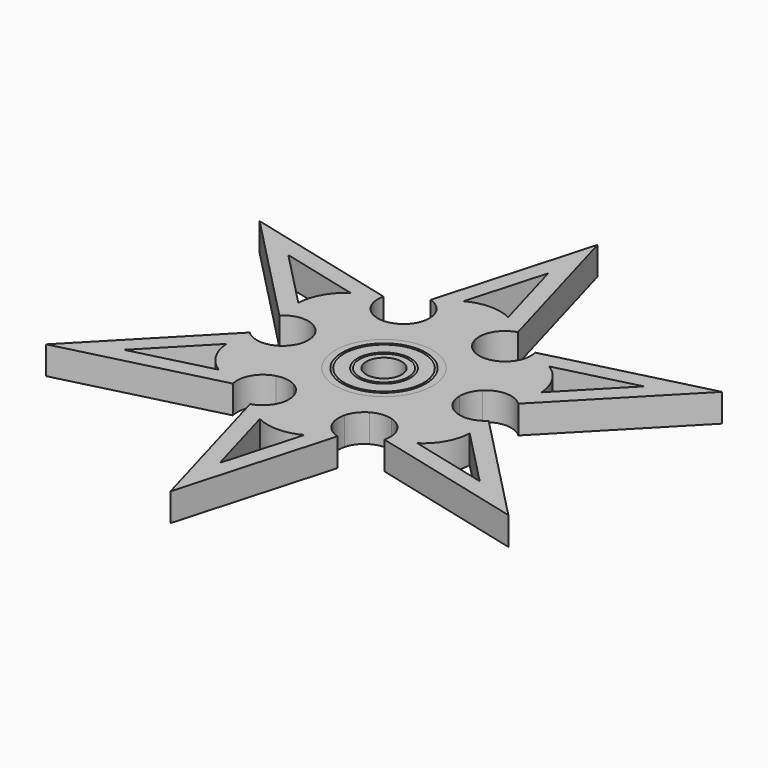
from build123d import *

# Parameters (mm, degrees)
F1_R     = 11
F1_R_2   = 4
F2_DEPTH = 6.35
F5_R     = 11
F6_DEPTH = 6.35
F8_DEPTH = 25.4


with BuildPart() as f2:
    # F1 (on Top) → F2 (new body)
    with BuildSketch(Plane.XY):
        Circle(F1_R)
        Circle(F1_R_2, mode=Mode.SUBTRACT)
    extrude(amount=F2_DEPTH)

    # F3 (on Right) → F4 (revolve, cut)
    with BuildSketch(Plane.YZ):
        with BuildLine():
            ThreePointArc((6, 6.35), (5.75, 6.6), (5.5, 6.35))
            Line((5.5, 6.35), (5.75, 6.35))
            Line((5.75, 6.35), (6, 6.35))
        make_face()
        with BuildLine():
            ThreePointArc((9.5, 6.35), (9.25, 6.6), (9, 6.35))
            Line((9, 6.35), (9.25, 6.35))
            Line((9.25, 6.35), (9.5, 6.35))
        make_face()
        with BuildLine():
            Line((9.25, 6.35), (9, 6.35))
            ThreePointArc((9, 6.35), (9.25, 6.1), (9.5, 6.35))
            Line((9.5, 6.35), (9.25, 6.35))
        make_face()
        with BuildLine():
            Line((5.75, 6.35), (5.5, 6.35))
            ThreePointArc((5.5, 6.35), (5.75, 6.1), (6, 6.35))
            Line((6, 6.35), (5.75, 6.35))
        make_face()
    revolve(axis=Axis((0, 0, 3.175), (0, 0, 1)), mode=Mode.SUBTRACT)


with BuildPart() as f6:
    # F5 (on Top) → F6 (new body)
    with BuildSketch(Plane.XY):
        with BuildLine():
            Line((0, 60.5), (0, 17.0180425354))
            Line((0, 17.0180425354), (5.8258503254, 18.4893295859))
            ThreePointArc((5.8258503254, 18.4893295859), (6.4320296551, 22.8503868027), (9.9057263273, 25.5558821098))
            Line((9.9057263273, 25.5558821098), (0, 60.5))
        make_face()
        with BuildLine():
            Line((-5.8258503254, 18.4893295859), (0, 17.0180425354))
            Line((0, 17.0180425354), (0, 60.5))
            Line((0, 60.5), (-9.9057263273, 25.5558821098))
            ThreePointArc((-9.9057263273, 25.5558821098), (-6.4320296551, 22.8503868027), (-5.8258503254, 18.4893295859))
        make_face()
        with BuildLine():
            Line((-18.9251542831, 4.1993304125), (-14.7380571583, 8.5090212677))
            Line((-14.7380571583, 8.5090212677), (-13.0993039576, 14.2899991734))
            ThreePointArc((-13.0993039576, 14.2899991734), (-16.5730006299, 16.9954944805), (-17.1791799596, 21.3565516973))
            Line((-17.1791799596, 21.3565516973), (-52.394536929, 30.25))
            Line((-52.394536929, 30.25), (-27.0849062869, 4.1993304125))
            ThreePointArc((-27.0849062869, 4.1993304125), (-23.005030285, 5.8548923222), (-18.9251542831, 4.1993304125))
        make_face()
        with BuildLine():
            Line((-13.0993039576, -14.2899991734), (-14.7380571583, -8.5090212677))
            Line((-14.7380571583, -8.5090212677), (-18.9251542831, -4.1993304125))
            ThreePointArc((-18.9251542831, -4.1993304125), (-23.005030285, -5.8548923222), (-27.0849062869, -4.1993304125))
            Line((-27.0849062869, -4.1993304125), (-52.394536929, -30.25))
            Line((-52.394536929, -30.25), (-17.1791799596, -21.3565516973))
            ThreePointArc((-17.1791799596, -21.3565516973), (-16.5730006299, -16.9954944805), (-13.0993039576, -14.2899991734))
        make_face()
        with BuildLine():
            Line((5.8258503254, -18.4893295859), (0, -17.0180425354))
            Line((0, -17.0180425354), (-5.8258503254, -18.4893295859))
            ThreePointArc((-5.8258503254, -18.4893295859), (-6.4320296551, -22.8503868027), (-9.9057263273, -25.5558821098))
            Line((-9.9057263273, -25.5558821098), (0, -60.5))
            Line((0, -60.5), (9.9057263273, -25.5558821098))
            ThreePointArc((9.9057263273, -25.5558821098), (6.4320296551, -22.8503868027), (5.8258503254, -18.4893295859))
        make_face()
        with BuildLine():
            Line((18.9251542831, -4.1993304125), (14.7380571583, -8.5090212677))
            Line((14.7380571583, -8.5090212677), (13.0993039576, -14.2899991734))
            ThreePointArc((13.0993039576, -14.2899991734), (16.5730006299, -16.9954944805), (17.1791799596, -21.3565516973))
            Line((17.1791799596, -21.3565516973), (52.394536929, -30.25))
            Line((52.394536929, -30.25), (27.0849062869, -4.1993304125))
            ThreePointArc((27.0849062869, -4.1993304125), (23.005030285, -5.8548923222), (18.9251542831, -4.1993304125))
        make_face()
        with BuildLine():
            Line((13.0993039576, 14.2899991734), (14.7380571583, 8.5090212677))
            Line((14.7380571583, 8.5090212677), (18.9251542831, 4.1993304125))
            ThreePointArc((18.9251542831, 4.1993304125), (23.005030285, 5.8548923222), (27.0849062869, 4.1993304125))
            Line((27.0849062869, 4.1993304125), (52.394536929, 30.25))
            Line((52.394536929, 30.25), (17.1791799596, 21.3565516973))
            ThreePointArc((17.1791799596, 21.3565516973), (16.5730006299, 16.9954944805), (13.0993039576, 14.2899991734))
        make_face()
        with BuildLine():
            ThreePointArc((15.8745077989, 4.5000002382), (16.3428788572, 2.2716317174), (16.5, 0))
            ThreePointArc((16.5, 0), (16.3428788623, -2.2716316803), (15.8745078193, -4.5000001663))
            Line((15.8745078193, -4.5000001663), (17.1501379628, 0))
            Line((17.1501379628, 0), (15.8745077989, 4.5000002382))
        make_face()
        with BuildLine():
            ThreePointArc((4.0401396495, 15.9977270764), (8.2500001412, 14.2894190809), (11.8343684535, 11.4977268756))
            Line((11.8343684535, 11.4977268756), (8.5750689814, 14.8524551542))
            Line((8.5750689814, 14.8524551542), (4.0401396495, 15.9977270764))
        make_face()
        with BuildLine():
            ThreePointArc((-11.8343682103, 11.4977271259), (-8.249999909, 14.289419215), (-4.0401394678, 15.9977271223))
            Line((-4.0401394678, 15.9977271223), (-8.5750689814, 14.8524551542))
            Line((-8.5750689814, 14.8524551542), (-11.8343682103, 11.4977271259))
        make_face()
        with BuildLine():
            Line((-17.1501379628, 0), (-15.8745078556, -4.5000000379))
            ThreePointArc((-15.8745078556, -4.5000000379), (-16.5, -4.12e-08), (-15.8745078781, 4.4999999586))
            Line((-15.8745078781, 4.4999999586), (-17.1501379628, 0))
        make_face()
        with BuildLine():
            Line((-8.5750689814, -14.8524551542), (-4.0401397191, -15.9977270589))
            ThreePointArc((-4.0401397191, -15.9977270589), (-8.2500001243, -14.2894190907), (-11.8343683762, -11.4977269552))
            Line((-11.8343683762, -11.4977269552), (-8.5750689814, -14.8524551542))
        make_face()
        with BuildLine():
            Line((8.5750689814, -14.8524551542), (11.8343682034, -11.4977271331))
            ThreePointArc((11.8343682034, -11.4977271331), (8.2500000987, -14.2894191055), (4.0401399023, -15.9977270126))
            Line((4.0401399023, -15.9977270126), (8.5750689814, -14.8524551542))
        make_face()
        with BuildLine():
            Line((14.7380571583, -8.5090212677), (11.8343682034, -11.4977271331))
            Line((11.8343682034, -11.4977271331), (8.5750689814, -14.8524551542))
            ThreePointArc((8.5750689814, -14.8524551542), (10.780191513, -14.1127760417), (13.0993039576, -14.2899991734))
            Line((13.0993039576, -14.2899991734), (14.7380571583, -8.5090212677))
        make_face()
        with BuildLine():
            Line((8.5750689814, -14.8524551542), (4.0401399023, -15.9977270126))
            Line((4.0401399023, -15.9977270126), (0, -17.0180425354))
            Line((0, -17.0180425354), (5.8258503254, -18.4893295859))
            ThreePointArc((5.8258503254, -18.4893295859), (6.8319268135, -16.3923077288), (8.5750689814, -14.8524551542))
        make_face()
        with BuildLine():
            Line((14.7380571583, 8.5090212677), (15.8745077989, 4.5000002382))
            Line((15.8745077989, 4.5000002382), (17.1501379628, 0))
            ThreePointArc((17.1501379628, 0), (17.6121183265, 2.2795316871), (18.9251542831, 4.1993304125))
            Line((18.9251542831, 4.1993304125), (14.7380571583, 8.5090212677))
        make_face()
        with BuildLine():
            Line((17.1501379628, 0), (15.8745078193, -4.5000001663))
            Line((15.8745078193, -4.5000001663), (14.7380571583, -8.5090212677))
            Line((14.7380571583, -8.5090212677), (18.9251542831, -4.1993304125))
            ThreePointArc((18.9251542831, -4.1993304125), (17.6121183265, -2.2795316871), (17.1501379628, 0))
        make_face()
        with BuildLine():
            Line((8.5750689814, 14.8524551542), (11.8343684535, 11.4977268756))
            Line((11.8343684535, 11.4977268756), (14.7380571583, 8.5090212677))
            Line((14.7380571583, 8.5090212677), (13.0993039576, 14.2899991734))
            ThreePointArc((13.0993039576, 14.2899991734), (10.780191513, 14.1127760417), (8.5750689814, 14.8524551542))
        make_face()
        with BuildLine():
            Line((-14.7380571583, 8.5090212677), (-11.8343682103, 11.4977271259))
            Line((-11.8343682103, 11.4977271259), (-8.5750689814, 14.8524551542))
            ThreePointArc((-8.5750689814, 14.8524551542), (-10.780191513, 14.1127760417), (-13.0993039576, 14.2899991734))
            Line((-13.0993039576, 14.2899991734), (-14.7380571583, 8.5090212677))
        make_face()
        with BuildLine():
            Line((-4.0401394678, 15.9977271223), (0, 17.0180425354))
            Line((0, 17.0180425354), (-5.8258503254, 18.4893295859))
            ThreePointArc((-5.8258503254, 18.4893295859), (-6.8319268135, 16.3923077288), (-8.5750689814, 14.8524551542))
            Line((-8.5750689814, 14.8524551542), (-4.0401394678, 15.9977271223))
        make_face()
        with BuildLine():
            Line((-14.7380571583, -8.5090212677), (-15.8745078556, -4.5000000379))
            Line((-15.8745078556, -4.5000000379), (-17.1501379628, 0))
            ThreePointArc((-17.1501379628, 0), (-17.6121183265, -2.2795316871), (-18.9251542831, -4.1993304125))
            Line((-18.9251542831, -4.1993304125), (-14.7380571583, -8.5090212677))
        make_face()
        with BuildLine():
            Line((-17.1501379628, 0), (-15.8745078781, 4.4999999586))
            Line((-15.8745078781, 4.4999999586), (-14.7380571583, 8.5090212677))
            Line((-14.7380571583, 8.5090212677), (-18.9251542831, 4.1993304125))
            ThreePointArc((-18.9251542831, 4.1993304125), (-17.6121183265, 2.2795316871), (-17.1501379628, 0))
        make_face()
        with BuildLine():
            Line((0, -17.0180425354), (-4.0401397191, -15.9977270589))
            Line((-4.0401397191, -15.9977270589), (-8.5750689814, -14.8524551542))
            ThreePointArc((-8.5750689814, -14.8524551542), (-6.8319268135, -16.3923077288), (-5.8258503254, -18.4893295859))
            Line((-5.8258503254, -18.4893295859), (0, -17.0180425354))
        make_face()
        with BuildLine():
            Line((-8.5750689814, -14.8524551542), (-11.8343683762, -11.4977269552))
            Line((-11.8343683762, -11.4977269552), (-14.7380571583, -8.5090212677))
            Line((-14.7380571583, -8.5090212677), (-13.0993039576, -14.2899991734))
            ThreePointArc((-13.0993039576, -14.2899991734), (-10.780191513, -14.1127760417), (-8.5750689814, -14.8524551542))
        make_face()
        with BuildLine():
            ThreePointArc((15.8745078193, -4.5000001663), (16.3428788623, -2.2716316803), (16.5, 0))
            ThreePointArc((16.5, 0), (16.3428788572, 2.2716317174), (15.8745077989, 4.5000002382))
            ThreePointArc((15.8745077989, 4.5000002382), (14.2894191735, 8.2499999809), (11.8343684535, 11.4977268756))
            ThreePointArc((11.8343684535, 11.4977268756), (8.2500001412, 14.2894190809), (4.0401396495, 15.9977270764))
            ThreePointArc((4.0401396495, 15.9977270764), (2.0356206963, 16.3739502986), (0, 16.5))
            ThreePointArc((0, 16.5), (-2.0356206033, 16.3739503102), (-4.0401394678, 15.9977271223))
            ThreePointArc((-4.0401394678, 15.9977271223), (-8.249999909, 14.289419215), (-11.8343682103, 11.4977271259))
            ThreePointArc((-11.8343682103, 11.4977271259), (-14.2894191589, 8.2500000062), (-15.8745078781, 4.4999999586))
            ThreePointArc((-15.8745078781, 4.4999999586), (-16.5, -4.12e-08), (-15.8745078556, -4.5000000379))
            ThreePointArc((-15.8745078556, -4.5000000379), (-14.2894191978, -8.2499999388), (-11.8343683762, -11.4977269552))
            ThreePointArc((-11.8343683762, -11.4977269552), (-8.2500001243, -14.2894190907), (-4.0401397191, -15.9977270589))
            ThreePointArc((-4.0401397191, -15.9977270589), (9.45e-08, -16.5), (4.0401399023, -15.9977270126))
            ThreePointArc((4.0401399023, -15.9977270126), (8.2500000987, -14.2894191055), (11.8343682034, -11.4977271331))
            ThreePointArc((11.8343682034, -11.4977271331), (14.2894191024, -8.2500001039), (15.8745078193, -4.5000001663))
        make_face()
        Circle(F5_R, mode=Mode.SUBTRACT)
        with BuildLine():
            ThreePointArc((-15.8745078781, 4.4999999586), (-14.2894191589, 8.2500000062), (-11.8343682103, 11.4977271259))
            Line((-11.8343682103, 11.4977271259), (-14.7380571583, 8.5090212677))
            Line((-14.7380571583, 8.5090212677), (-15.8745078781, 4.4999999586))
        make_face()
        with BuildLine():
            ThreePointArc((-4.0401394678, 15.9977271223), (-2.0356206033, 16.3739503102), (0, 16.5))
            Line((0, 16.5), (0, 17.0180425354))
            Line((0, 17.0180425354), (-4.0401394678, 15.9977271223))
        make_face()
        with BuildLine():
            ThreePointArc((0, 16.5), (2.0356206963, 16.3739502986), (4.0401396495, 15.9977270764))
            Line((4.0401396495, 15.9977270764), (0, 17.0180425354))
            Line((0, 17.0180425354), (0, 16.5))
        make_face()
        with BuildLine():
            Line((0, 17.0180425354), (4.0401396495, 15.9977270764))
            Line((4.0401396495, 15.9977270764), (8.5750689814, 14.8524551542))
            ThreePointArc((8.5750689814, 14.8524551542), (6.8319268135, 16.3923077288), (5.8258503254, 18.4893295859))
            Line((5.8258503254, 18.4893295859), (0, 17.0180425354))
        make_face()
        with BuildLine():
            Line((-14.7380571583, -8.5090212677), (-11.8343683762, -11.4977269552))
            ThreePointArc((-11.8343683762, -11.4977269552), (-14.2894191978, -8.2499999388), (-15.8745078556, -4.5000000379))
            Line((-15.8745078556, -4.5000000379), (-14.7380571583, -8.5090212677))
        make_face()
        with BuildLine():
            Line((0, -17.0180425354), (4.0401399023, -15.9977270126))
            ThreePointArc((4.0401399023, -15.9977270126), (9.45e-08, -16.5), (-4.0401397191, -15.9977270589))
            Line((-4.0401397191, -15.9977270589), (0, -17.0180425354))
        make_face()
        with BuildLine():
            Line((14.7380571583, -8.5090212677), (15.8745078193, -4.5000001663))
            ThreePointArc((15.8745078193, -4.5000001663), (14.2894191024, -8.2500001039), (11.8343682034, -11.4977271331))
            Line((11.8343682034, -11.4977271331), (14.7380571583, -8.5090212677))
        make_face()
        with BuildLine():
            ThreePointArc((11.8343684535, 11.4977268756), (14.2894191735, 8.2499999809), (15.8745077989, 4.5000002382))
            Line((15.8745077989, 4.5000002382), (14.7380571583, 8.5090212677))
            Line((14.7380571583, 8.5090212677), (11.8343684535, 11.4977268756))
        make_face()
    extrude(amount=F6_DEPTH)

    # F7 (on face) → F8 (cut)
    with BuildSketch(Plane.XY.offset(6.35)):
        with BuildLine():
            ThreePointArc((27.4652588739, -10.0584216992), (26.0836032425, -15.0120346435), (22.6012069234, -18.7962346069))
            Line((22.6012069234, -18.7962346069), (40.2961620381, -23.265))
            Line((40.2961620381, -23.265), (27.4652588739, -10.0584216992))
        make_face()
        with BuildLine():
            ThreePointArc((5.0217807235, -28.814822756), (0.0409982575, -30.095080352), (-4.9774132034, -28.9713366553))
            Line((-4.9774132034, -28.9713366553), (0, -46.53))
            Line((0, -46.53), (5.0217807235, -28.814822756))
        make_face()
        with BuildLine():
            ThreePointArc((-22.4434781505, -18.7564010567), (-26.042604985, -15.0830457085), (-27.5786201268, -10.1751020484))
            Line((-27.5786201268, -10.1751020484), (-40.2961620381, -23.265))
            Line((-40.2961620381, -23.265), (-22.4434781505, -18.7564010567))
        make_face()
        with BuildLine():
            ThreePointArc((-27.4652588739, 10.0584216992), (-26.0836032425, 15.0120346435), (-22.6012069234, 18.7962346069))
            Line((-22.6012069234, 18.7962346069), (-40.2961620381, 23.265))
            Line((-40.2961620381, 23.265), (-27.4652588739, 10.0584216992))
        make_face()
        with BuildLine():
            ThreePointArc((-5.0217807235, 28.814822756), (-0.0409982575, 30.095080352), (4.9774132034, 28.9713366553))
            Line((4.9774132034, 28.9713366553), (0, 46.53))
            Line((0, 46.53), (-5.0217807235, 28.814822756))
        make_face()
        with BuildLine():
            ThreePointArc((22.4434781505, 18.7564010567), (26.042604985, 15.0830457085), (27.5786201268, 10.1751020484))
            Line((27.5786201268, 10.1751020484), (40.2961620381, 23.265))
            Line((40.2961620381, 23.265), (22.4434781505, 18.7564010567))
        make_face()
    extrude(amount=-F8_DEPTH, mode=Mode.SUBTRACT)


solid = Compound([f2.part, f6.part])
